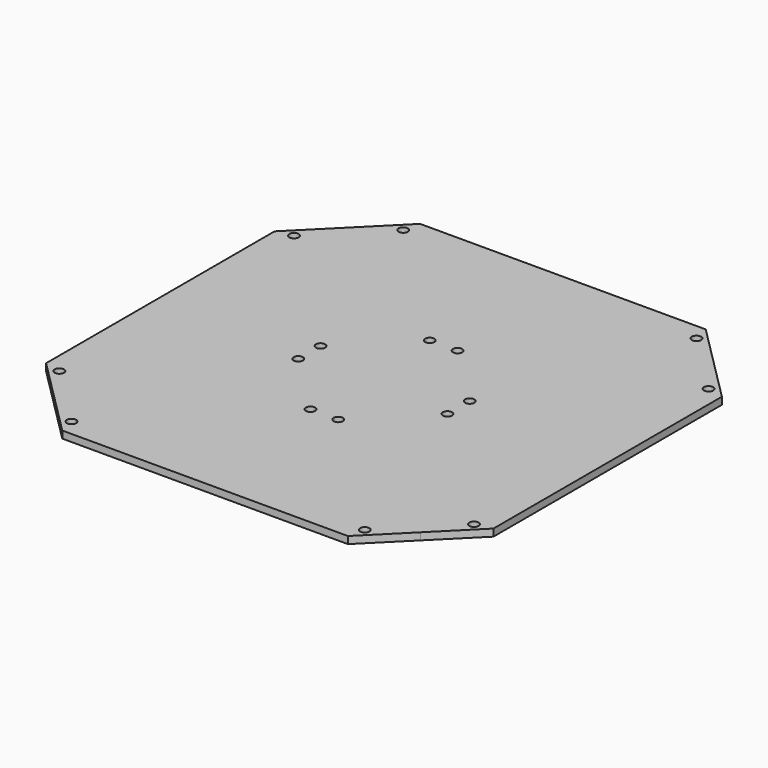
from build123d import *

# Parameters (mm, degrees)
F1_DEPTH = 4
F2_R     = 2.6
F3_DEPTH = 20
F4_R     = 2.6
F5_DEPTH = 4.001


# Not quite as in the source:
# - a feature names something its author has since deleted; it is built from what else it names


with BuildPart() as f1:
    # F0 (on Top) → F1 (new body)
    with BuildSketch(Plane.XY):
        Polygon((125.15, 79.85), (102.5, 102.5), (79.85, 125.15), (-79.9109665441, 125.15), (-102.530483272, 102.530483272), (-125.15, 79.9109665441), (-125.15, -79.85), (-102.5, -102.5), (-79.85, -125.15), (79.9109665441, -125.15), (102.530483272, -102.530483272), (125.15, -79.9109665441), align=None)
    extrude(amount=F1_DEPTH)

    # F2 (on face) → F3 (cut)
    with BuildSketch(Plane.XY.offset(4)):
        with Locations((-7.7781745931, 41.71930009)):
            Circle(F2_R)
        with Locations((-41.71930009, 7.7781745931)):
            Circle(F2_R)
        with Locations((7.7781745931, -41.71930009)):
            Circle(F2_R)
        with Locations((41.71930009, -7.7781745931)):
            Circle(F2_R)
        with Locations((41.71930009, 7.7781745931)):
            Circle(F2_R)
        with Locations((7.7781745931, 41.71930009)):
            Circle(F2_R)
        with Locations((-41.71930009, -7.7781745931)):
            Circle(F2_R)
        with Locations((-7.7781745931, -41.71930009)):
            Circle(F2_R)
    extrude(amount=-F3_DEPTH, mode=Mode.SUBTRACT)

    # F4 (on face) → F5 (cut, through all)
    with BuildSketch(Plane.XY.offset(4)):
        with Locations((-82.0243866176, 115.9655121146)):
            Circle(F4_R)
        with Locations((-115.9655121146, 82.0243866176)):
            Circle(F4_R)
        with Locations((82.0243866176, -115.9655121146)):
            Circle(F4_R)
        with Locations((115.9655121146, -82.0243866176)):
            Circle(F4_R)
        with Locations((82.0243866176, 115.9655121146)):
            Circle(F4_R)
        with Locations((115.9655121146, 82.0243866176)):
            Circle(F4_R)
        with Locations((-115.9655121146, -82.0243866176)):
            Circle(F4_R)
        with Locations((-82.0243866176, -115.9655121146)):
            Circle(F4_R)
    extrude(amount=-F5_DEPTH, mode=Mode.SUBTRACT)


solid = f1.part
